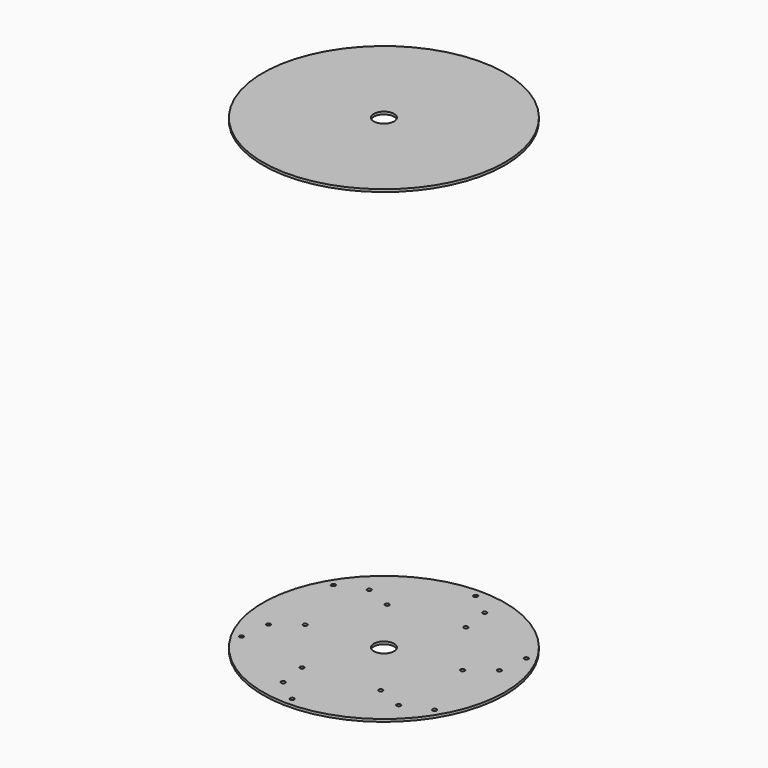
from build123d import *

# Parameters (mm, degrees)
F0_R     = 301.625
F0_R_2   = 25.4
F1_DEPTH = 6.35
F5_R     = 301.625
F5_R_2   = 25.4
F7_DEPTH = 6.35
F6_R     = 5.08
F8_DEPTH = 6.351


# Not quite as in the source:
# - the program builds the solid bodies; features that only make, move or delete a surface that nothing else refers to are left out


with BuildPart() as f1:
    # F0 (on Top) → F1 (new body)
    with BuildSketch(Plane.XY):
        Circle(F0_R)
        Circle(F0_R_2, mode=Mode.SUBTRACT)
    extrude(amount=F1_DEPTH)

    # F6 (on face) → F8 (cut, through all)
    with BuildSketch(Plane.XY.offset(6.35)):
        with BuildLine():
            Line((-240.46551283, 138.8328285632), (-245.9224430153, 141.9833886746))
            ThreePointArc((-245.9224430153, 141.9833886746), (-243.7414687643, 139.4598266645), (-240.46551283, 138.8328285632))
        make_face()
        with BuildLine():
            ThreePointArc((-236.1214687643, 143.8592357157), (-242.1564166176, 148.8486720163), (-245.9224430153, 141.9833886746))
            Line((-245.9224430153, 141.9833886746), (-240.46551283, 138.8328285632))
            ThreePointArc((-240.46551283, 138.8328285632), (-237.3579641041, 140.5375084652), (-236.1214687643, 143.8592357157))
        make_face()
        with Locations((-174.1461598977, 171.7307498537)):
            Circle(F6_R)
        with Locations((-107.9254532481, 144.8362073709)):
            Circle(F6_R)
        with Locations((-245.186487081, -136.9569815221)):
            Circle(F6_R)
        with Locations((-235.7962719331, -64.949623516)):
            Circle(F6_R)
        with Locations((-179.394561595, -21.0480805423)):
            Circle(F6_R)
        with BuildLine():
            ThreePointArc((0, -277.6656571265), (-9.0650183167, -280.8162172379), (0, -283.9667773493))
            Line((0, -283.9667773493), (0, -277.6656571265))
        make_face()
        with BuildLine():
            Line((0, -277.6656571265), (0, -283.9667773493))
            ThreePointArc((0, -283.9667773493), (0.8134341968, -282.4839262879), (1.0949816833, -280.8162172379))
            ThreePointArc((1.0949816833, -280.8162172379), (0.8134341968, -279.1485081878), (0, -277.6656571265))
        make_face()
        with Locations((-61.6501120354, -236.6803733697)):
            Circle(F6_R)
        with Locations((-71.469108347, -165.8842879132)):
            Circle(F6_R)
        with Locations((107.9254532481, -144.8362073709)):
            Circle(F6_R)
        with Locations((174.1461598977, -171.7307498537)):
            Circle(F6_R)
        with Locations((241.2014687643, -143.8592357157)):
            Circle(F6_R)
        with Locations((179.394561595, 21.0480805423)):
            Circle(F6_R)
        with Locations((235.7962719331, 64.949623516)):
            Circle(F6_R)
        with BuildLine():
            Line((240.46551283, 138.8328285632), (245.9224430153, 141.9833886746))
            ThreePointArc((245.9224430153, 141.9833886746), (242.646487081, 141.3563905734), (240.46551283, 138.8328285632))
        make_face()
        with BuildLine():
            ThreePointArc((250.266487081, 136.9569815221), (249.0299917412, 140.2787087727), (245.9224430153, 141.9833886746))
            Line((245.9224430153, 141.9833886746), (240.46551283, 138.8328285632))
            ThreePointArc((240.46551283, 138.8328285632), (244.2315392277, 131.9675452216), (250.266487081, 136.9569815221))
        make_face()
        with Locations((71.469108347, 165.8842879132)):
            Circle(F6_R)
        with Locations((61.6501120354, 236.6803733697)):
            Circle(F6_R)
        with Locations((3.9850183167, 280.8162172379)):
            Circle(F6_R)
    extrude(amount=-F8_DEPTH, mode=Mode.SUBTRACT)


with BuildPart() as f7:
    # F5 (on offset) → F7 (new body)
    with BuildSketch(Plane.XY.offset(1162.05)):
        Circle(F5_R)
        Circle(F5_R_2, mode=Mode.SUBTRACT)
    extrude(amount=F7_DEPTH)


solid = Compound([f1.part, f7.part])
